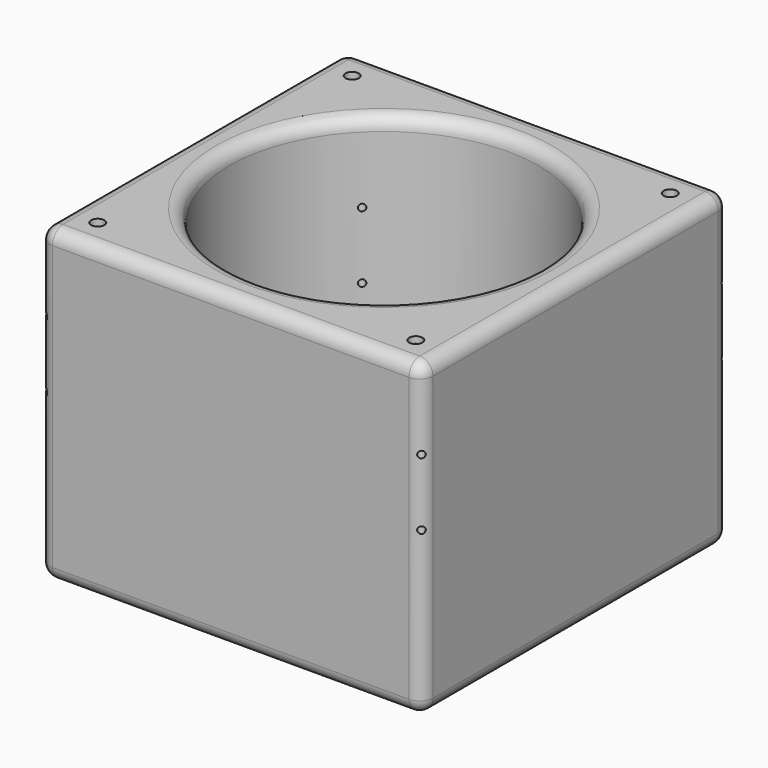
from build123d import *

# Parameters (mm, degrees)
F0_W            = 288
F0_H            = 288
F0_R            = 116.5
F1_DEPTH        = 233
F2_R            = 10
F7_D            = 5.1
F7_DEPTH        = 203.6477529817
F8_D            = 5.1
F9_D            = 5.1
F9_DEPTH        = 203.6477531231
F10_D           = 5.1
F12_D           = 5.1
F12_CBORE_D     = 10
F12_CBORE_DEPTH = 5
F14_DEPTH       = 5


with BuildPart() as f1:
    # F0 (on Top) → F1 (new body)
    with BuildSketch(Plane.XY):
        Rectangle(F0_W, F0_H)
        Circle(F0_R, mode=Mode.SUBTRACT)
    extrude(amount=F1_DEPTH)

    # F2
    f2_edges = [f1.edges().sort_by_distance(p)[0] for p in [
        (144, 0, 233),
        (0, 144, 233),
        (-144, 0, 233),
        (0, -144, 233),
        (-116.5, 0, 233),
        (144, 0, 0),
        (0, 144, 0),
        (-144, 0, 0),
        (0, -144, 0),
        (-116.5, 0, 0),
        (-144, 144, 116.5),
        (-144, -144, 116.5),
        (144, -144, 116.5),
        (144, 144, 116.5),
    ]]
    fillet(f2_edges, radius=F2_R)

    # F7 (through all, one way)
    with BuildSketch(Plane(origin=(0, 0, 0), x_dir=(0.7071067812, 0.7071067812, 0), z_dir=(0.7071067812, -0.7071067812, 0))):
        with Locations((0, 173), (0, 123)):
            Circle(F7_D / 2)
    extrude(amount=-F7_DEPTH, mode=Mode.SUBTRACT)

    # F8 (through all)
    with Locations(Plane(origin=(0, 0, 0), x_dir=(0.7071067812, 0.7071067812, 0), z_dir=(-0.7071067812, 0.7071067812, 0))):
        with Locations((0, -173), (0, -123)):
            Hole(F8_D / 2)

    # F9 (through all, one way)
    with BuildSketch(Plane(origin=(0, 0, 0), x_dir=(-0.7071067812, 0.7071067812, 0), z_dir=(0.7071067812, 0.7071067812, 0))):
        with Locations((0, 173), (0, 123)):
            Circle(F9_D / 2)
    extrude(amount=-F9_DEPTH, mode=Mode.SUBTRACT)

    # F10 (through all)
    with Locations(Plane(origin=(0, 0, 0), x_dir=(-0.7071067812, 0.7071067812, 0), z_dir=(-0.7071067812, -0.7071067812, 0))):
        with Locations((0, -173), (0, -123)):
            Hole(F10_D / 2)

    # F12 (through all)
    with Locations(Plane.XY.offset(233)):
        with Locations((-119.5364013596, -119.5364013596), (119.5364013596, -119.5364013596), (119.5364013596, 119.5364013596), (-119.5364013596, 119.5364013596)):
            CounterBoreHole(F12_D / 2, F12_CBORE_D / 2, F12_CBORE_DEPTH)

    # F13 (on face) → F14 (cut)
    with BuildSketch(Plane.XY):
        Polygon((-124.5364013596, 116.6496500136), (-119.5364013596, 113.7628986677), (-119.5364013596, 119.5364013596), (-114.5364013596, 119.5364013596), (-114.5364013596, 122.4231527055), (-119.5364013596, 125.3099040515), (-124.5364013596, 122.4231527055), align=None)
        Polygon((-119.5364013596, 119.5364013596), (-119.5364013596, 113.7628986677), (-114.5364013596, 116.6496500136), (-114.5364013596, 119.5364013596), align=None)
        Polygon((114.5364013596, 116.6496500136), (119.5364013596, 113.7628986677), (119.5364013596, 119.5364013596), (114.5364013596, 119.5364013596), align=None)
        Polygon((119.5364013596, 119.5364013596), (119.5364013596, 113.7628986677), (124.5364013596, 116.6496500136), (124.5364013596, 122.4231527055), (119.5364013596, 125.3099040515), (114.5364013596, 122.4231527055), (114.5364013596, 119.5364013596), align=None)
        Polygon((114.5364013596, -119.5364013596), (119.5364013596, -119.5364013596), (119.5364013596, -113.7628986677), (114.5364013596, -116.6496500136), align=None)
        Polygon((119.5364013596, -113.7628986677), (119.5364013596, -119.5364013596), (114.5364013596, -119.5364013596), (114.5364013596, -122.4231527055), (119.5364013596, -125.3099040515), (124.5364013596, -122.4231527055), (124.5364013596, -116.6496500136), align=None)
        Polygon((-119.5364013596, -119.5364013596), (-114.5364013596, -119.5364013596), (-114.5364013596, -116.6496500136), (-119.5364013596, -113.7628986677), align=None)
        Polygon((-114.5364013596, -122.4231527055), (-114.5364013596, -119.5364013596), (-119.5364013596, -119.5364013596), (-119.5364013596, -113.7628986677), (-124.5364013596, -116.6496500136), (-124.5364013596, -122.4231527055), (-119.5364013596, -125.3099040515), align=None)
    extrude(amount=F14_DEPTH, mode=Mode.SUBTRACT)


solid = f1.part
